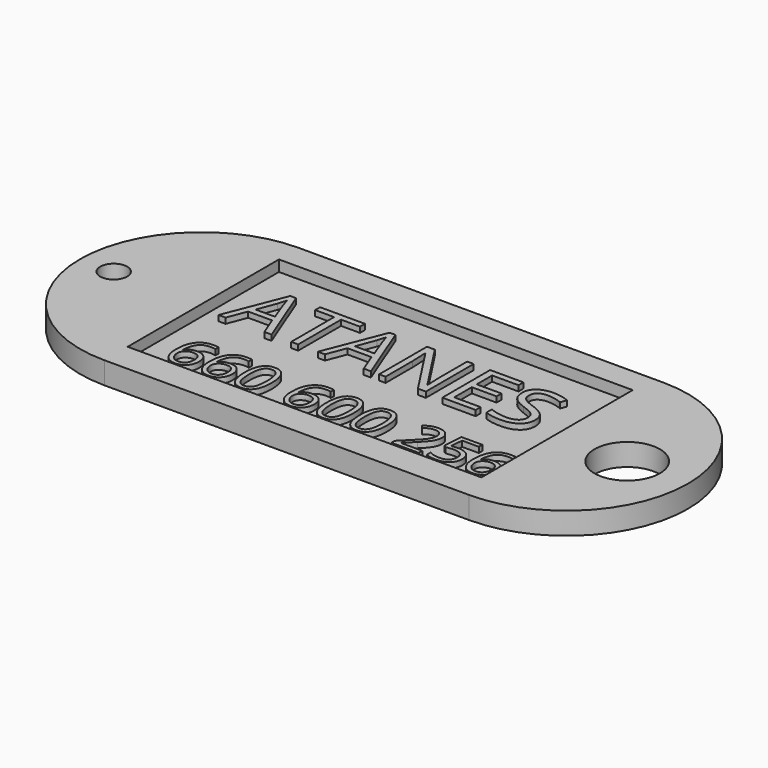
from build123d import *

# Parameters (mm, degrees)
F0_R           = 1.2175240656
F0_R_2         = 2.9606075995
F1_DEPTH       = 2
F2_W           = 32
F2_H           = 17.1107510105
F3_DEPTH       = 1
F4_TEXT_SIZE   = 7.5784487863
F4_TEXT_SIZE_2 = 5.2805280528
F5_DEPTH       = 0.5


# Not quite as in the source:
# - Text() gives the source's letters only with a copy of the font that has no kerning and outlines rounded to 1/6400 em; it was checked with that copy


with BuildPart() as f1:
    # F0 (on Top) → F1 (new body)
    with BuildSketch(Plane.XY):
        with BuildLine():
            ThreePointArc((16.5, -11), (27.5, 0), (16.5, 11))
            Line((16.5, 11), (-16.5, 11))
            ThreePointArc((-16.5, 11), (-27.5, 0), (-16.5, -11))
            Line((-16.5, -11), (16.5, -11))
        make_face()
        with Locations((-24.4516190141, 0)):
            Circle(F0_R, mode=Mode.SUBTRACT)
        Polygon((0, -7.9586589709), (-16.5, -7.9586589709), (-16.5, 7.973828353), (0, 7.973828353), (16.5, 7.973828353), (16.5, -7.9586589709), align=None, mode=Mode.SUBTRACT)
        with Locations((22, 0)):
            Circle(F0_R_2, mode=Mode.SUBTRACT)
        Polygon((-16.5, 7.973828353), (-16.5, -7.9586589709), (0, -7.9586589709), (16.5, -7.9586589709), (16.5, 7.973828353), (0, 7.973828353), align=None)
    extrude(amount=F1_DEPTH)

    # F2 (on face) → F3 (cut)
    with BuildSketch(Plane.XY.offset(2)):
        with Locations((-0.5, 0.1915735193)):
            Rectangle(F2_W, F2_H)
    extrude(amount=-F3_DEPTH, mode=Mode.SUBTRACT)

    # F4 (on face) → F5 (join)
    with BuildSketch(Plane.XY.offset(1)):
        with Locations((-15.1230813935, 0.1915735193)):
            Text('ATANES', F4_TEXT_SIZE, font='Open Sans', text_align=(TextAlign.LEFT, TextAlign.BOTTOM))
        with Locations((-14.5, -7.4377400192)):
            Text('660 600 256', F4_TEXT_SIZE_2, font='Open Sans', text_align=(TextAlign.LEFT, TextAlign.BOTTOM))
    extrude(amount=F5_DEPTH)


solid = f1.part
